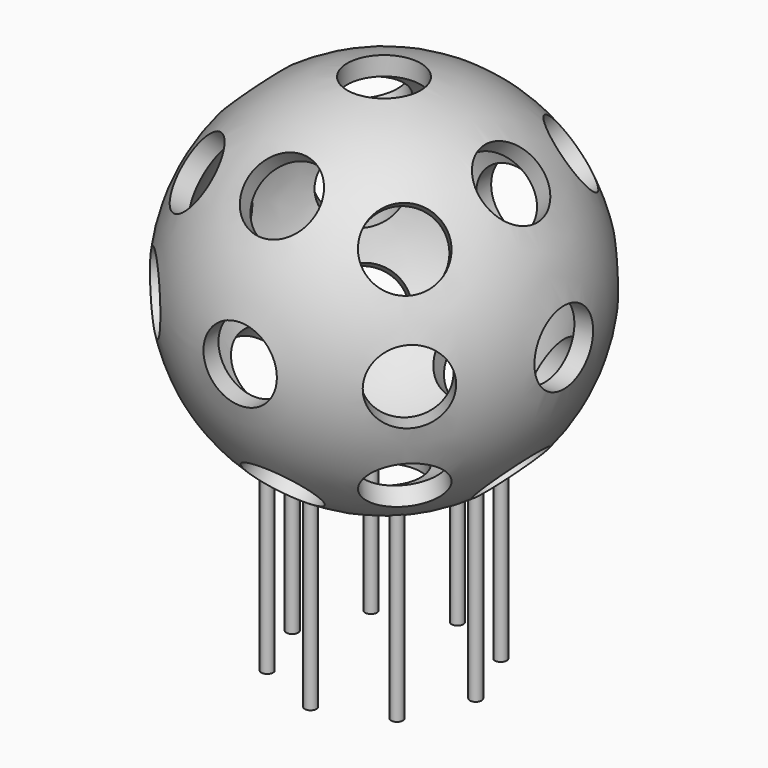
from build123d import *

# Parameters (mm, degrees)
F22_R            = 2.54
F23_DEPTH        = 38.1
F25_R            = 2.54
F26_DEPTH        = 38.1
F28_R            = 2.54
F29_DEPTH        = 38.1
F31_R            = 2.54
F32_DEPTH        = 127
F34_R            = 2.54
F35_DEPTH        = 127
F37_R            = 2.54
F38_DEPTH        = 127
F40_R            = 2.54
F41_DEPTH        = 127
F54_R            = 2.54
F55_DEPTH        = 63.5
F61_R            = 2.54
F62_DEPTH        = 63.5
F62_COPIES_COUNT = 3
F62_COPIES_ANGLE = 180
F69_R            = 2.54
F70_DEPTH        = 50.8
F73_R            = 2.54
F74_DEPTH        = 12.4444079933
F76_R            = 0.4064
F77_DEPTH        = 12.7
F77_COPIES_COUNT = 8


# Not quite as in the source:
# - a pattern or mirror of a feature is missing from the dataset's text; its kind, count and spacing are read off the source's solid


with BuildPart() as f2:
    # F1 (on Top) → F2 (revolve)
    with BuildSketch(Plane.XY):
        with BuildLine():
            Line((0, -12.7), (0, 12.7))
            ThreePointArc((0, 12.7), (-12.7, 0), (0, -12.7))
        make_face()
    revolve(axis=Axis((0, 0, 0), (0, -1, 0)))

    # F22 (on plane+point) → F23 (cut, symmetric)
    with BuildSketch(Plane.XY.offset(12.7)):
        Circle(F22_R)
    f23 = extrude(amount=F23_DEPTH, both=True, mode=Mode.SUBTRACT)

    # F23_copies: F23 across plane
    add(f23.mirror(Plane(origin=(0, 0, 0), x_dir=(0, 0.3843930227, -0.9231695424), z_dir=(0, -0.9231695424, -0.3843930227))), mode=Mode.SUBTRACT)

    # F25 (on plane+point) → F26 (cut, symmetric)
    with BuildSketch(Plane.YZ.offset(12.7)):
        Circle(F25_R)
    extrude(amount=F26_DEPTH, both=True, mode=Mode.SUBTRACT)

    # F28 (on plane+point) → F29 (cut, symmetric)
    with BuildSketch(Plane.XZ.offset(-12.7)):
        Circle(F28_R)
    extrude(amount=F29_DEPTH, both=True, mode=Mode.SUBTRACT)

    # F31 (on plane+point) → F32 (cut, symmetric)
    with BuildSketch(Plane(origin=(7.3323484187, -7.3323484187, 7.3323484187), x_dir=(-0.8164965809, -0.4082482905, 0.4082482905), z_dir=(-0.5773502692, 0.5773502692, -0.5773502692))):
        Circle(F31_R)
    extrude(amount=F32_DEPTH, both=True, mode=Mode.SUBTRACT)

    # F34 (on plane+point) → F35 (cut, symmetric)
    with BuildSketch(Plane(origin=(-7.3323484187, 7.3323484187, 7.3323484187), x_dir=(-0.8164965809, -0.4082482905, -0.4082482905), z_dir=(-0.5773502692, 0.5773502692, 0.5773502692))):
        Circle(F34_R)
    extrude(amount=F35_DEPTH, both=True, mode=Mode.SUBTRACT)

    # F37 (on plane+point) → F38 (cut, symmetric)
    with BuildSketch(Plane(origin=(7.3323484187, 7.3323484187, 7.3323484187), x_dir=(0.8164965809, -0.4082482905, -0.4082482905), z_dir=(-0.5773502692, -0.5773502692, -0.5773502692))):
        Circle(F37_R)
    extrude(amount=F38_DEPTH, both=True, mode=Mode.SUBTRACT)

    # F40 (on plane+point) → F41 (cut, symmetric)
    with BuildSketch(Plane(origin=(7.3323484187, 7.3323484187, -7.3323484187), x_dir=(-0.8164965809, 0.4082482905, -0.4082482905), z_dir=(0.5773502692, 0.5773502692, -0.5773502692))):
        Circle(F40_R)
    extrude(amount=F41_DEPTH, both=True, mode=Mode.SUBTRACT)

    # F42 (on Top) → F43 (revolve, cut)
    with BuildSketch(Plane.XY):
        with BuildLine():
            Line((0, -11.43), (0, 11.43))
            ThreePointArc((0, 11.43), (-11.43, 0), (0, -11.43))
        make_face()
    revolve(axis=Axis((0, 6.35, 0), (0, 1, 0)), mode=Mode.SUBTRACT)

    # F54 (on face) → F55 (cut, symmetric)
    with BuildSketch(Plane(origin=(0, 8.3731673765, 8.4353982834), x_dir=(1, 0, 0), z_dir=(0, -0.7044840082, -0.7097198618))):
        Circle(F54_R)
    extrude(amount=F55_DEPTH, both=True, mode=Mode.SUBTRACT)

    # F61 (on 3pt) → F62 (cut, symmetric)
    with BuildSketch(Plane(origin=(7.3323484187, 0, 7.3323484187), x_dir=(0.7071067812, 0, -0.7071067812), z_dir=(-0.7071067812, 0, -0.7071067812))):
        Circle(F61_R)
    f62 = extrude(amount=F62_DEPTH, both=True, mode=Mode.SUBTRACT)

    # F62_copies: F62 ×3 about axis
    f62_copies_axis = Axis((0, 0, 0), (1, 0, 0))
    for i in range(1, F62_COPIES_COUNT):
        add(f62.rotate(f62_copies_axis, i * F62_COPIES_ANGLE / (F62_COPIES_COUNT - 1)), mode=Mode.SUBTRACT)

    # F69 (on 3pt) → F70 (cut, symmetric)
    with BuildSketch(Plane(origin=(-7.3323484187, -7.3323484187, 0), x_dir=(0.7071067812, -0.7071067812, 0), z_dir=(-0.7071067812, -0.7071067812, 0))):
        Circle(F69_R)
    extrude(amount=F70_DEPTH, both=True, mode=Mode.SUBTRACT)

    # F73 (on Top) → F74 (cut, through all)
    with BuildSketch(Plane.XY):
        Circle(F73_R)
    extrude(amount=-F74_DEPTH, mode=Mode.SUBTRACT)

    # F76 (on offset) → F77 (join)
    with BuildSketch(Plane.XY.offset(-10.668)):
        with Locations((0, -6.35)):
            Circle(F76_R)
    f77 = extrude(amount=-F77_DEPTH)

    # F77_copies: F77 ×8 about axis
    f77_copies_axis = Axis((0, 0, 0), (0, 0, 1))
    for i in range(1, F77_COPIES_COUNT):
        add(f77.rotate(f77_copies_axis, i * 360 / F77_COPIES_COUNT))


solid = f2.part
